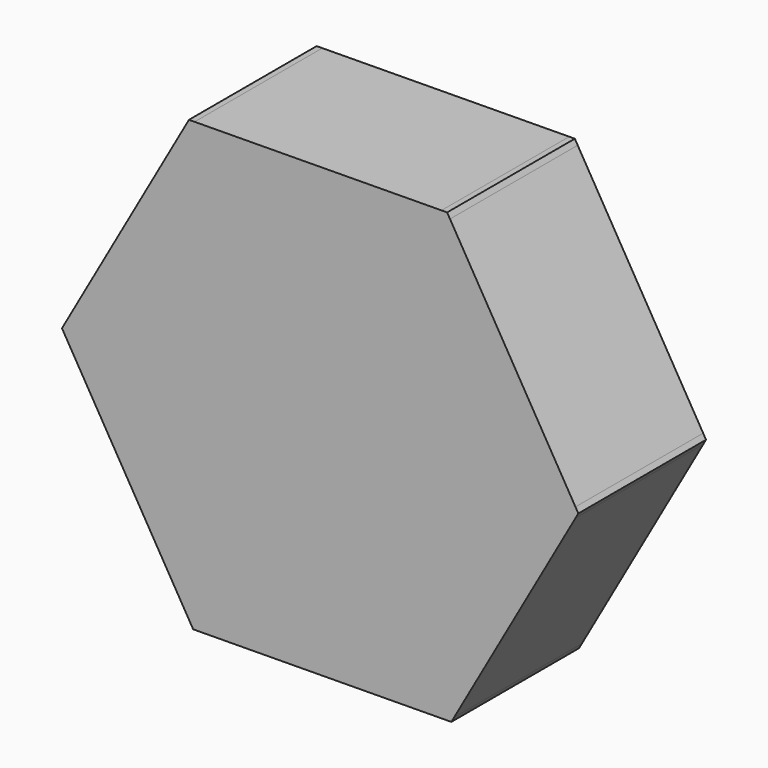
from build123d import *

# Parameters (mm, degrees)
F1_DEPTH = 25


with BuildPart() as f1:
    # F0 (on Front) → F1 (new body)
    with BuildSketch(Plane.XZ):
        with BuildLine():
            ThreePointArc((-12.9923656989, 28.902602186), (-12.9909523706, 29.0967337225), (-12.9904812574, 29.290869832))
            ThreePointArc((-12.9904812574, 29.290869832), (-12.9945641617, 29.8623728238), (-13.0068120409, 30.4337591459))
            Line((-13.0068120409, 30.4337591459), (-32.6551738333, 63.7361201862))
            ThreePointArc((-32.6551738333, 63.7361201862), (-33.3181920134, 64.1190342382), (-33.9884178287, 64.489187767))
            Line((-33.9884178287, 64.489187767), (-72.6532893918, 64.1243878322))
            ThreePointArc((-72.6532893918, 64.1243878322), (-73.3164117783, 63.741654271), (-73.9720870452, 63.3462984531))
            Line((-73.9720870452, 63.3462984531), (-92.988596816, 29.679137478))
            ThreePointArc((-92.988596816, 29.679137478), (-92.9887010223, 28.9134898649), (-92.974150474, 28.1479805181))
            Line((-92.974150474, 28.1479805181), (-73.3257886816, -5.1543805222))
            ThreePointArc((-73.3257886816, -5.1543805222), (-72.6627705014, -5.5372945741), (-71.9925446861, -5.9074481029))
            Line((-71.9925446861, -5.9074481029), (-33.3276731231, -5.5426481682))
            ThreePointArc((-33.3276731231, -5.5426481682), (-32.6645507366, -5.1599146069), (-32.0088754696, -4.764558789))
            Line((-32.0088754696, -4.764558789), (-12.9923656989, 28.902602186))
        make_face()
        with BuildLine():
            ThreePointArc((-13.0068120409, 30.4337591459), (-12.9945641617, 29.8623728238), (-12.9904812574, 29.290869832))
            ThreePointArc((-12.9904812574, 29.290869832), (-12.9909523706, 29.0967337225), (-12.9923656989, 28.902602186))
            Line((-12.9923656989, 28.902602186), (-12.5575819284, 29.6723509657))
            Line((-12.5575819284, 29.6723509657), (-13.0068120409, 30.4337591459))
        make_face()
        with BuildLine():
            ThreePointArc((-33.9884178287, 64.489187767), (-33.3181920134, 64.1190342382), (-32.6551738333, 63.7361201862))
            Line((-32.6551738333, 63.7361201862), (-33.1044039458, 64.4975283665))
            Line((-33.1044039458, 64.4975283665), (-33.9884178287, 64.489187767))
        make_face()
        with BuildLine():
            Line((-32.4436592401, -5.5343075687), (-32.0088754696, -4.764558789))
            ThreePointArc((-32.0088754696, -4.764558789), (-32.6645507366, -5.1599146069), (-33.3276731231, -5.5426481682))
            Line((-33.3276731231, -5.5426481682), (-32.4436592401, -5.5343075687))
        make_face()
        with BuildLine():
            ThreePointArc((-73.9720870452, 63.3462984531), (-73.3164117783, 63.741654271), (-72.6532893918, 64.1243878322))
            Line((-72.6532893918, 64.1243878322), (-73.5373032748, 64.1160472328))
            Line((-73.5373032748, 64.1160472328), (-73.9720870452, 63.3462984531))
        make_face()
        with BuildLine():
            Line((-72.8765585691, -5.9157887024), (-71.9925446861, -5.9074481029))
            ThreePointArc((-71.9925446861, -5.9074481029), (-72.6627705014, -5.5372945741), (-73.3257886816, -5.1543805222))
            Line((-73.3257886816, -5.1543805222), (-72.8765585691, -5.9157887024))
        make_face()
        with BuildLine():
            ThreePointArc((-92.974150474, 28.1479805181), (-92.9887010223, 28.9134898649), (-92.988596816, 29.679137478))
            Line((-92.988596816, 29.679137478), (-93.4233805865, 28.9093886984))
            Line((-93.4233805865, 28.9093886984), (-92.974150474, 28.1479805181))
        make_face()
    extrude(amount=F1_DEPTH)


solid = f1.part
